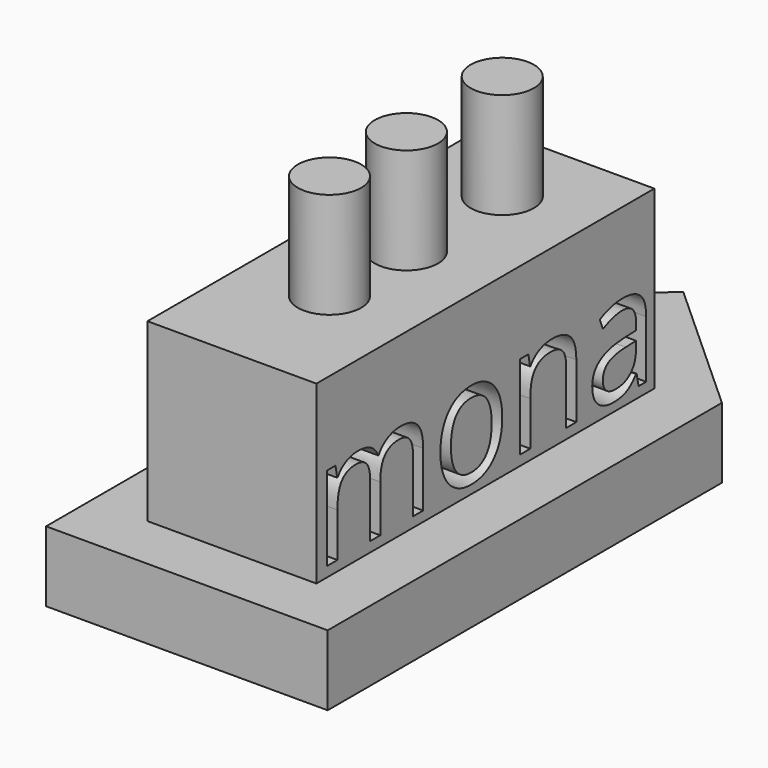
from build123d import *

# Parameters (mm, degrees)
F1_DEPTH     = 10
F2_W         = 24
F2_H         = 60
F3_DEPTH     = 25
F4_R         = 4.5
F5_DEPTH     = 15
F6_TEXT_SIZE = 10.9797330677
F7_DEPTH     = 5
F8_TEXT_SIZE = 22.3216880777
F9_DEPTH     = 5


# Not quite as in the source:
# - Text() gives the source's letters only with a copy of the font that has no kerning and outlines rounded to 1/6400 em; it was checked with that copy


with BuildPart() as f1:
    # F0 (on Top) → F1 (new body)
    with BuildSketch(Plane.XY):
        Polygon((-39.0050960092, 58.7321769812), (-59.0050960092, 40.593819834), (-59.0050960092, -29.406180166), (-19.0050960092, -29.406180166), (-19.0050960092, 40.593819834), align=None)
    extrude(amount=F1_DEPTH)

    # F2 (on face) → F3 (join)
    with BuildSketch(Plane.XY.offset(10)):
        with Locations((-39.0050960092, 8.593819834)):
            Rectangle(F2_W, F2_H)
    extrude(amount=F3_DEPTH)

    # F4 (on face) → F5 (join)
    with BuildSketch(Plane.XY.offset(35)):
        with Locations((-39.0050960092, 26.5911162514)):
            Circle(F4_R)
        with Locations((-39.0050960092, 9.5667902652)):
            Circle(F4_R)
        with Locations((-39.0050960092, -4.0820221809)):
            Circle(F4_R)
    extrude(amount=F5_DEPTH)

    # F6 (on face) → F7 (cut)
    with BuildSketch(Plane(origin=(-51.0050960092, 0, 0), x_dir=(0, -1, 0), z_dir=(-1, 0, 0))):
        with Locations((-31.0135148466, 15.6081086025)):
            Text('manal', F6_TEXT_SIZE, font='Open Sans', text_align=(TextAlign.LEFT, TextAlign.BOTTOM))
    extrude(amount=-F7_DEPTH, mode=Mode.SUBTRACT)

    # F8 (on face) → F9 (cut)
    with BuildSketch(Plane.YZ.offset(-27.0050960092)):
        with Locations((-21.406180166, 11.4236536197)):
            Text('mona', F8_TEXT_SIZE, font='Open Sans', text_align=(TextAlign.LEFT, TextAlign.BOTTOM))
    extrude(amount=-F9_DEPTH, mode=Mode.SUBTRACT)


solid = f1.part
